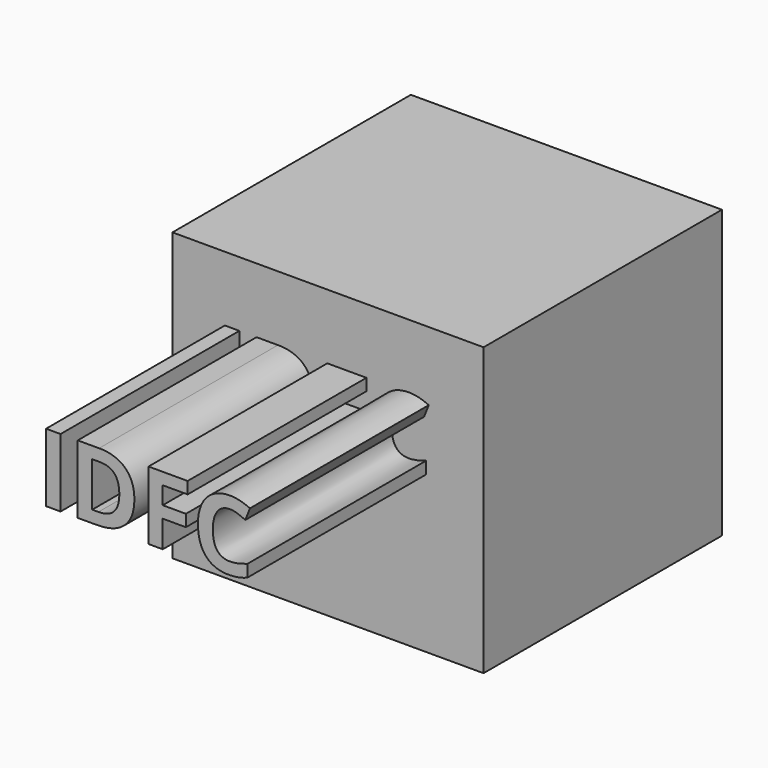
from build123d import *

# Parameters (mm, degrees)
F0_W         = 106.0703992844
F0_H         = 97.8407971561
F1_DEPTH     = 101.6
F2_TEXT_SIZE = 32.5966678146
F3_DEPTH     = 76.2


# Not quite as in the source:
# - Text() gives the source's letters only with a copy of the font that has no kerning and outlines rounded to 1/6400 em; it was checked with that copy


with BuildPart() as f1:
    # F0 (on Front) → F1 (new body)
    with BuildSketch(Plane.XZ):
        with Locations((3.0479989946, 4.8767980188)):
            Rectangle(F0_W, F0_H)
    extrude(amount=F1_DEPTH)

    # F2 (on face) → F3 (join)
    with BuildSketch(Plane.XZ.offset(101.6)):
        with Locations((-35.0520014763, 8.3820000291)):
            Text('IDFC', F2_TEXT_SIZE, font='Open Sans', font_style=FontStyle.BOLD, text_align=(TextAlign.LEFT, TextAlign.BOTTOM))
    extrude(amount=F3_DEPTH)


solid = f1.part
